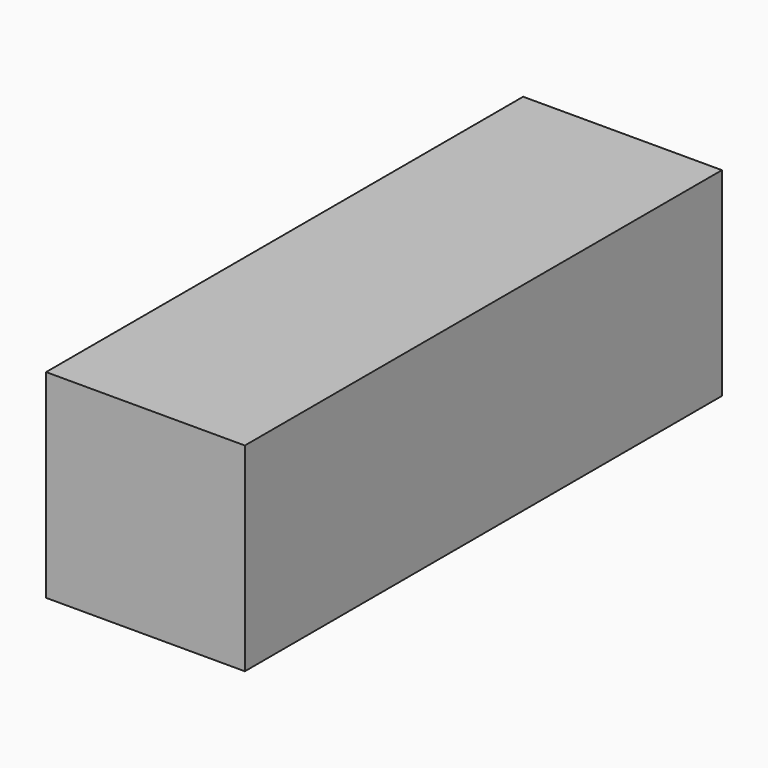
from build123d import *

# Parameters (mm, degrees)
F0_W     = 6.35
F0_H     = 6.35
F1_DEPTH = 19.05


# Not quite as in the source:
# - a length typed as a fraction of an inch, garbled in the dataset ("3 / 203.2 mm" for 3/8 in), is restored


with BuildPart() as f1:
    # F0 (on Front) → F1 (new body)
    with BuildSketch(Plane.XZ):
        with Locations((3.175, 3.175)):
            Rectangle(F0_W, F0_H)
    extrude(amount=F1_DEPTH)


solid = f1.part
